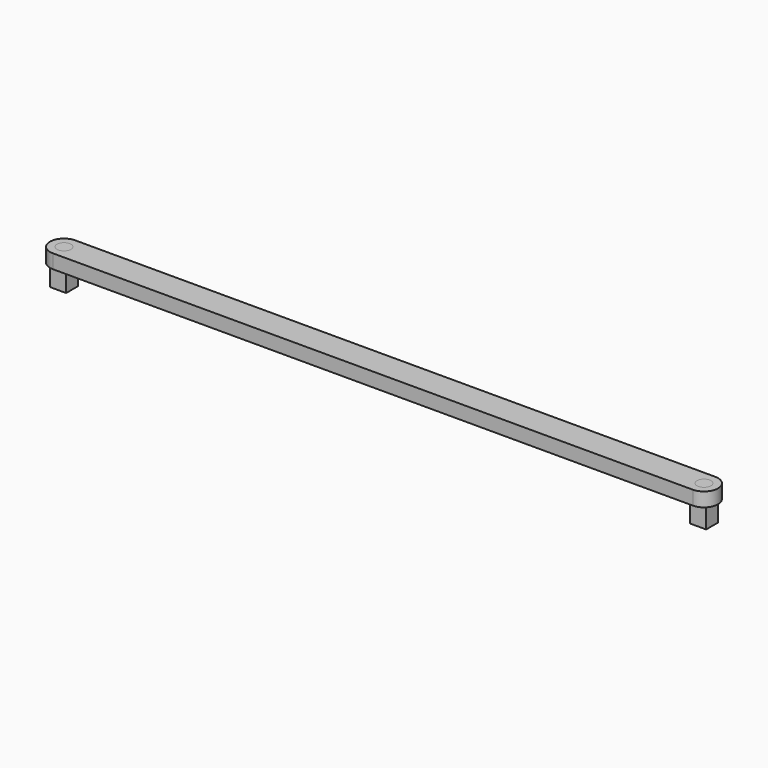
from build123d import *

# Parameters (mm, degrees)
F0_R     = 5
F1_DEPTH = 10
F2_W     = 11.6554063559
F2_H     = 10.7572656125
F3_DEPTH = 15
F4_DEPTH = 10


with BuildPart() as f1:
    # F0 (on Top) → F1 (new body)
    with BuildSketch(Plane.XY):
        with BuildLine():
            Line((475.696013391, 54.4301785901), (18.696013391, 54.4301785901))
            ThreePointArc((18.696013391, 54.4301785901), (8.696013391, 44.4301785901), (18.696013391, 34.4301785901))
            Line((18.696013391, 34.4301785901), (475.696013391, 34.4301785901))
            ThreePointArc((475.696013391, 34.4301785901), (485.696013391, 44.4301785901), (475.696013391, 54.4301785901))
        make_face()
        with Locations((18.696013391, 44.4301785901)):
            Circle(F0_R, mode=Mode.SUBTRACT)
        with Locations((475.696013391, 44.4301785901)):
            Circle(F0_R, mode=Mode.SUBTRACT)
    extrude(amount=F1_DEPTH)


with BuildPart() as f3:
    # F2 (on Top) → F3 (new body)
    with BuildSketch(Plane.XY):
        with Locations((18.696013391, 44.4301785901)):
            Rectangle(F2_W, F2_H)
    extrude(amount=-F3_DEPTH)

    # F0 (on Top) → F4 (join)
    with BuildSketch(Plane.XY):
        with Locations((18.696013391, 44.4301785901)):
            Circle(F0_R)
    extrude(amount=F4_DEPTH)


with BuildPart() as f3b:
    # F2 (on Top) → F3, piece 2 (new body)
    with BuildSketch(Plane.XY):
        with Locations((475.696013391, 44.4301785901)):
            Rectangle(F2_W, F2_H)
    extrude(amount=-F3_DEPTH)

    # F0 (on Top) → F4, piece 2 (join)
    with BuildSketch(Plane.XY):
        with Locations((475.696013391, 44.4301785901)):
            Circle(F0_R)
    extrude(amount=F4_DEPTH)


solid = Compound([f1.part, f3.part, f3b.part])
